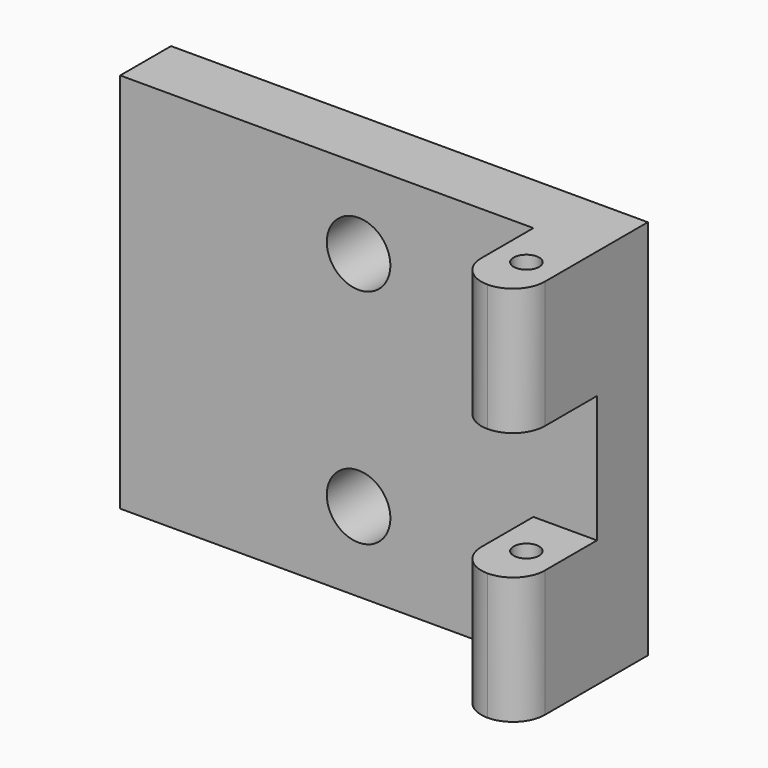
from build123d import *

# Parameters (mm, degrees)
F0_W     = 15
F0_H     = 12
F1_DEPTH = 2
F2_W     = 2
F2_H     = 4
F3_DEPTH = 3.05
F4_R     = 0.4
F5_DEPTH = 25
F6_R     = 0.99999
F7_R     = 1
F8_DEPTH = 25


# Not quite as in the source:
# - a fillet or chamfer is up to 0.001 mm smaller than in the source, because OpenCascade refuses the exact size


with BuildPart() as f1:
    # F0 (on Front) → F1 (new body)
    with BuildSketch(Plane.XZ):
        Rectangle(F0_W, F0_H)
    extrude(amount=F1_DEPTH)

    # F2 (on face) → F3 (join)
    with BuildSketch(Plane.XZ.offset(2)):
        with Locations((6.5, 4)):
            Rectangle(F2_W, F2_H)
        with Locations((6.5, -4)):
            Rectangle(F2_W, F2_H)
    extrude(amount=F3_DEPTH)

    # F4 (on face) → F5 (cut)
    with BuildSketch(Plane(origin=(0, 0, -6), x_dir=(1, 0, 0), z_dir=(0, 0, -1))):
        with Locations((6.5, 3.525)):
            Circle(F4_R)
    extrude(amount=-F5_DEPTH, mode=Mode.SUBTRACT)

    # F6 (radius 1 in the source; OpenCascade refuses exactly that, so slightly less here)
    f6_edges = [f1.edges().sort_by_distance(p)[0] for p in [
        (7.5, -5.05, 4),
        (5.5, -5.05, 4),
        (7.5, -5.05, -4),
        (5.5, -5.05, -4),
    ]]
    fillet(f6_edges, radius=F6_R)

    # F7 (on face) → F8 (cut)
    with BuildSketch(Plane(origin=(0, 0, 0), x_dir=(-1, 0, 0), z_dir=(0, 1, 0))):
        with Locations((0, 3.5)):
            Circle(F7_R)
        with Locations((0, -3.5)):
            Circle(F7_R)
    extrude(amount=-F8_DEPTH, mode=Mode.SUBTRACT)


solid = f1.part
